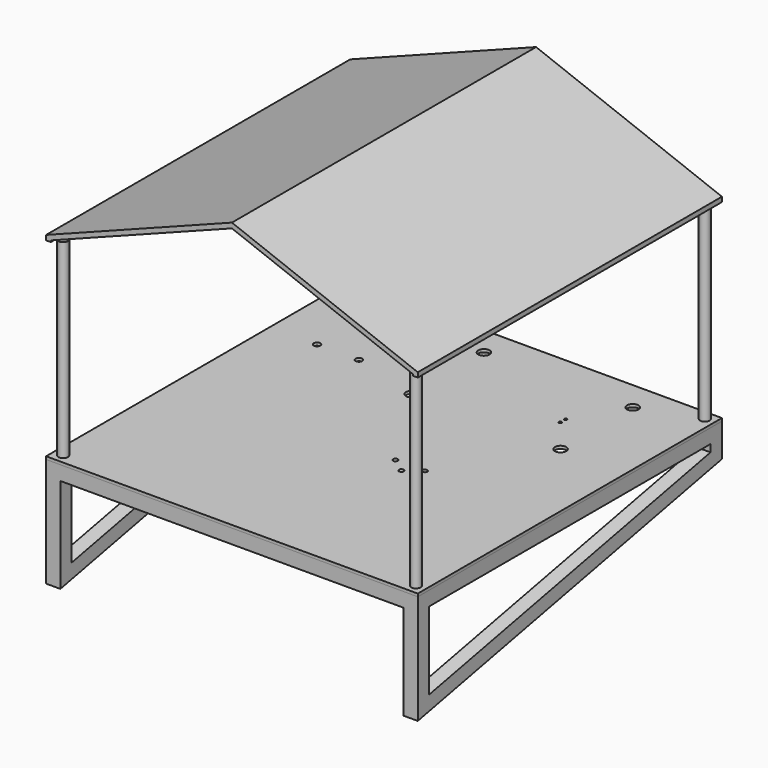
from build123d import *

# Parameters (mm, degrees)
F0_W      = 391.06
F0_H      = 400
F0_R      = 2.5
F0_R_2    = 3.5
F0_R_3    = 6
F0_R_4    = 1.5
F1_DEPTH  = 1.5
F2_W      = 391.06
F2_H      = 400
F2_W_2    = 361.06
F2_H_2    = 370
F3_DEPTH  = 15
F5_DEPTH  = 15
F7_R      = 5
F8_DEPTH  = 200
F9_W      = 391.06
F9_H      = 400
F10_DEPTH = 80
F12_DEPTH = 400
F13_T     = -5


with BuildPart() as f1:
    # F0 (on Top) → F1 (new body, symmetric)
    with BuildSketch(Plane.XY):
        Rectangle(F0_W, F0_H)
        with Locations((32.73, -25.9125)):
            Circle(F0_R, mode=Mode.SUBTRACT)
        with Locations((48.23, -37.5)):
            Circle(F0_R, mode=Mode.SUBTRACT)
        with Locations((63.73, -25.9125)):
            Circle(F0_R, mode=Mode.SUBTRACT)
        with Locations((-146.005, 94.449)):
            Circle(F0_R_2, mode=Mode.SUBTRACT)
        with Locations((-102.063, 94.449)):
            Circle(F0_R_2, mode=Mode.SUBTRACT)
        with Locations((-30.07, 74)):
            Circle(F0_R_3, mode=Mode.SUBTRACT)
        with Locations((-146.005, 148.551)):
            Circle(F0_R_2, mode=Mode.SUBTRACT)
        with Locations((-102.063, 148.551)):
            Circle(F0_R_2, mode=Mode.SUBTRACT)
        with Locations((-30.07, 169)):
            Circle(F0_R_3, mode=Mode.SUBTRACT)
        with Locations((126.53, 74)):
            Circle(F0_R_3, mode=Mode.SUBTRACT)
        with Locations((96.73, 111)):
            Circle(F0_R_4, mode=Mode.SUBTRACT)
        with Locations((96.73, 118)):
            Circle(F0_R_4, mode=Mode.SUBTRACT)
        with Locations((126.53, 169)):
            Circle(F0_R_3, mode=Mode.SUBTRACT)
    extrude(amount=F1_DEPTH, both=True)

    # F7 (on face) → F8 (join)
    with BuildSketch(Plane.XY.offset(1.5)):
        with Locations((-185.53, 190)):
            Circle(F7_R)
        with Locations((185.53, 190)):
            Circle(F7_R)
        with Locations((185.53, -190)):
            Circle(F7_R)
        with Locations((-185.53, -190)):
            Circle(F7_R)
    extrude(amount=F8_DEPTH)


with BuildPart() as f3:
    # F2 (on face) → F3 (new body)
    with BuildSketch(Plane(origin=(0, 0, -1.5), x_dir=(1, 0, 0), z_dir=(0, 0, -1))):
        Rectangle(F2_W, F2_H)
        Rectangle(F2_W_2, F2_H_2, mode=Mode.SUBTRACT)
    extrude(amount=F3_DEPTH)

    # F4 (on face) → F5 (join)
    with BuildSketch(Plane.YZ.offset(195.53)):
        Polygon((-185, -16.5), (-200, -16.5), (-200, -116.5), (200, -36.5), (200, -16.5), (185, -16.5), (185, -24.2029414592), (-185, -98.2029414592), align=None)
    extrude(amount=-F5_DEPTH)

    # F6: F3 across plane


with BuildPart() as f3_1:
    add(f3.part)
    add(f3.part.mirror(Plane.YZ))


with BuildPart() as f10:
    # F9 (on face) → F10 (new body)
    with BuildSketch(Plane.XY.offset(201.5)):
        Rectangle(F9_W, F9_H)
    extrude(amount=F10_DEPTH)

    # F11 (on face) → F12 (cut, through all)
    with BuildSketch(Plane.XZ.offset(200)):
        Polygon((-195.53, 281.5), (-195.53, 206.5), (0, 281.5), align=None)
        Polygon((195.53, 281.5), (0, 281.5), (195.53, 206.5), align=None)
    extrude(amount=-F12_DEPTH, mode=Mode.SUBTRACT)

    # F13
    f13_openings = [f10.faces().sort_by_distance(p)[0] for p in [
        (0, 0, 201.5),
        (0, 200, 228.264706),
        (0, -200, 228.264706),
    ]]
    offset(amount=F13_T, openings=f13_openings)


solid = Compound([f1.part, f3_1.part, f10.part])
